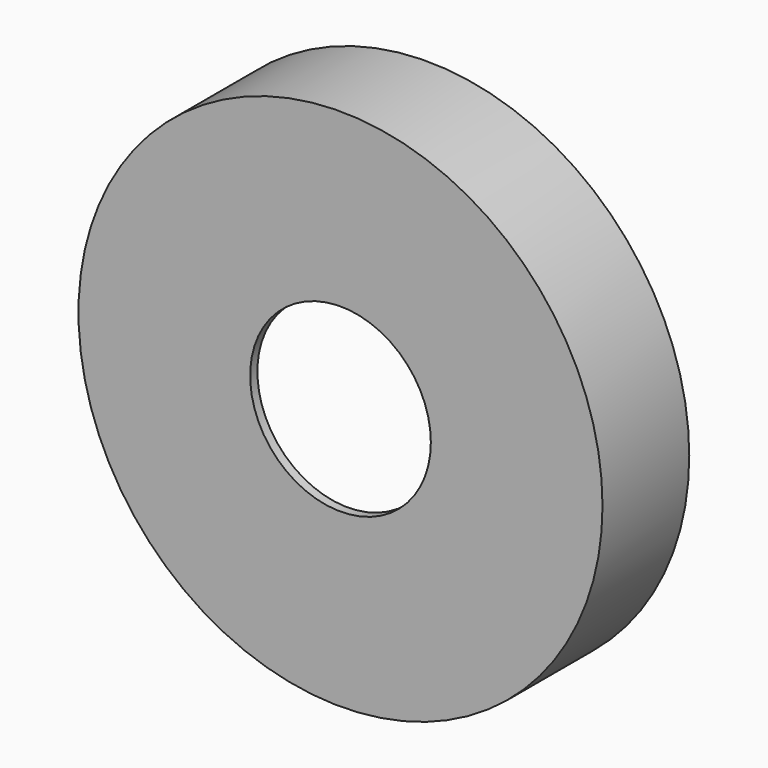
from build123d import *

# Parameters (mm, degrees)
F0_R     = 5.8
F1_DEPTH = 1.8
F2_R     = 5.8
F2_R_2   = 4.7
F3_DEPTH = 0.4
F4_R     = 4.7
F5_DEPTH = 1.8
F6_R     = 5.8
F6_R_2   = 4.7
F6_R_3   = 2
F7_DEPTH = 0.2


# Not quite as in the source:
# - a feature names something its author has since deleted; it is built from what else it names


with BuildPart() as f1:
    # F0 (on Front) → F1 (new body)
    with BuildSketch(Plane.XZ):
        Circle(F0_R)
    extrude(amount=F1_DEPTH)

    # F2 (on face) → F3 (join)
    with BuildSketch(Plane.XZ.offset(1.8)):
        Circle(F2_R)
        Circle(F2_R_2, mode=Mode.SUBTRACT)
    extrude(amount=F3_DEPTH)

    # F4 (on face) → F5 (cut)
    with BuildSketch(Plane.XZ.offset(1.8)):
        Circle(F4_R)
    extrude(amount=-F5_DEPTH, mode=Mode.SUBTRACT)

    # F6 (on face) → F7 (join)
    with BuildSketch(Plane.XZ.offset(2.2)):
        Circle(F6_R)
        Circle(F6_R_2, mode=Mode.SUBTRACT)
        Circle(F6_R_2)
        Circle(F6_R_3, mode=Mode.SUBTRACT)
    extrude(amount=F7_DEPTH)


solid = f1.part
